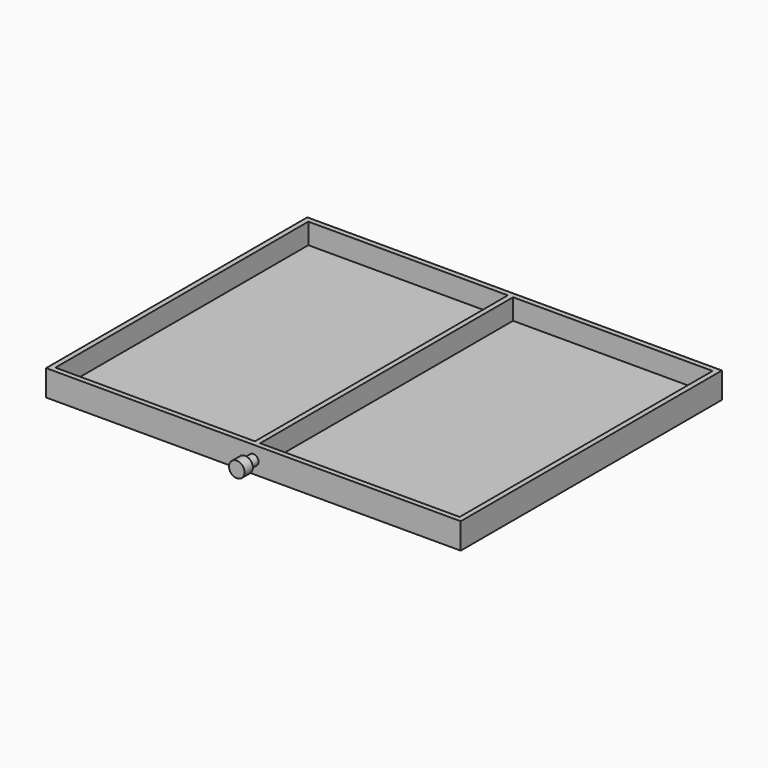
from build123d import *

# Parameters (mm, degrees)
F0_W      = 38.3663107641
F0_H      = 42.2096475959
F1_DEPTH  = 0.6858
F3_W      = 400
F3_H      = 305
F4_DEPTH  = 5
F5_W      = 5
F5_H      = 305
F6_DEPTH  = 20
F7_W      = 5
F7_H      = 305
F8_DEPTH  = 20
F9_W      = 400
F9_H      = 25
F10_DEPTH = 5
F11_W     = 5
F11_H     = 305
F12_DEPTH = 20
F13_W     = 400
F13_H     = 25
F14_DEPTH = 5
F15_R     = 5
F16_DEPTH = 10
F17_R     = 7.5
F17_R_2   = 5
F18_DEPTH = 10


with BuildPart() as f1:
    # F0 (on Top) → F1 (new body)
    with BuildSketch(Plane.XY):
        with Locations((-14.0401979443, 21.1048237979)):
            Rectangle(F0_W, F0_H)
    extrude(amount=F1_DEPTH)


with BuildPart() as f4:
    # F3 (on Top) → F4 (new body)
    with BuildSketch(Plane.XY):
        Rectangle(F3_W, F3_H)
    extrude(amount=F4_DEPTH)

    # F5 (on face) → F6 (join)
    with BuildSketch(Plane.XY.offset(5)):
        with Locations((-197.5, 0)):
            Rectangle(F5_W, F5_H)
    extrude(amount=F6_DEPTH)

    # F7 (on face) → F8 (join)
    with BuildSketch(Plane.XY.offset(5)):
        with Locations((197.5, 0)):
            Rectangle(F7_W, F7_H)
    extrude(amount=F8_DEPTH)

    # F9 (on face) → F10 (join)
    with BuildSketch(Plane(origin=(0, 152.5, 0), x_dir=(-1, 0, 0), z_dir=(0, 1, 0))):
        with Locations((0, 12.5)):
            Rectangle(F9_W, F9_H)
    extrude(amount=F10_DEPTH)

    # F11 (on face) → F12 (join)
    with BuildSketch(Plane.XY.offset(5)):
        Rectangle(F11_W, F11_H)
    extrude(amount=F12_DEPTH)

    # F13 (on face) → F14 (join)
    with BuildSketch(Plane.XZ.offset(152.5)):
        with Locations((0, 12.5)):
            Rectangle(F13_W, F13_H)
    extrude(amount=F14_DEPTH)

    # F15 (on face) → F16 (join)
    with BuildSketch(Plane.XZ.offset(157.5)):
        with Locations((0, 12.090690434)):
            Circle(F15_R)
    extrude(amount=F16_DEPTH)

    # F17 (on face) → F18 (join)
    with BuildSketch(Plane.XZ.offset(167.5)):
        with Locations((0, 12.090690434)):
            Circle(F17_R)
        with Locations((0, 12.090690434)):
            Circle(F17_R_2, mode=Mode.SUBTRACT)
        with Locations((0, 12.090690434)):
            Circle(F17_R_2)
    extrude(amount=F18_DEPTH)


solid = f4.part
